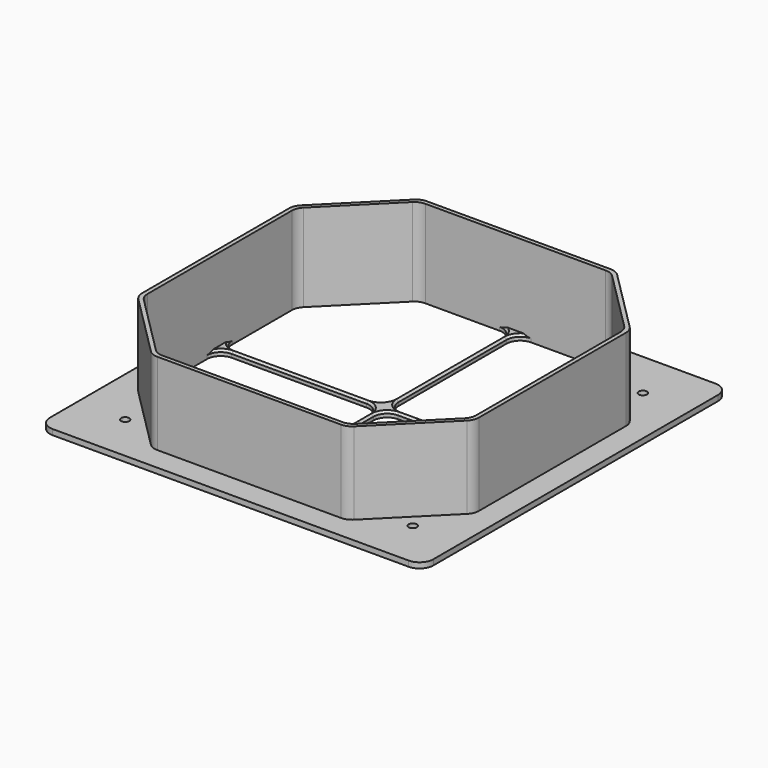
from build123d import *

# Parameters (mm, degrees)
F0_W         = 59.25
F0_H         = 1.5
F0_W_2       = 1.5
F0_H_2       = 59.25
F1_DEPTH     = 2
F0_W_3       = 140
F0_H_3       = 140
F2_DEPTH     = 32
F3_D         = 3
F4_R         = 5
F5_T1_DEPTH  = 49.25
F5_T3_DEPTH  = 49.25
F5_T5_DEPTH  = 49.25
F5_T7_DEPTH  = 49.25
F5_T12_ANGLE = 127.5884718038
F5_T15_ANGLE = 90
F5_T19_ANGLE = 127.5884718038
F5_T24_ANGLE = 127.5884718038
F5_T27_ANGLE = 90
F5_T31_ANGLE = 127.5884718038
F5_T36_ANGLE = 127.5884718038
F5_T39_ANGLE = 90
F5_T43_ANGLE = 127.5884718038
F5_T48_ANGLE = 127.5884718038
F5_T53_ANGLE = 127.5884718038
F5_T56_ANGLE = 90


# Not quite as in the source:
# - a fillet or chamfer that OpenCascade refuses, or shapes differently, is made with other operations: its cross-section is extruded or revolved along the edge and cut away or added


with BuildPart() as f1:
    # F0 (on Top) → F1 (new body)
    with BuildSketch(Plane.XY):
        with Locations((-36.375, 0)):
            Rectangle(F0_W, F0_H)
        with Locations((-6, 30.375)):
            Rectangle(F0_W_2, F0_H_2)
        with Locations((-6, -30.375)):
            Rectangle(F0_W_2, F0_H_2)
        with Locations((24.375, 0)):
            Rectangle(F0_W, F0_H)
        with Locations((-6, 0)):
            Rectangle(F0_W_2, F0_H)
    extrude(amount=F1_DEPTH)



with BuildPart() as f1b:
    # F0 (on Top) → F1, piece 2 (new body)
    with BuildSketch(Plane.XY):
        with Locations((-6, 0)):
            Rectangle(F0_W_3, F0_H_3)
        Polygon((55.5000009226, -35.6213207257), (29.6213207257, -61.5000009226), (-41.6213207257, -61.5000009226), (-67.5000009226, -35.6213207257), (-67.5000009226, 35.6213207257), (-41.6213207257, 61.5000009226), (29.6213207257, 61.5000009226), (55.5000009226, 35.6213207257), align=None, mode=Mode.SUBTRACT)
    extrude(amount=F1_DEPTH)


with BuildPart() as f1_1:
    add(f1.part)

    add(f1b.part)  # F2 merges F1b
    # F0 (on Top) → F2 (join)
    with BuildSketch(Plane.XY):
        Polygon((-41.6213207257, -61.5000009226), (29.6213207257, -61.5000009226), (55.5000009226, -35.6213207257), (55.5000009226, 35.6213207257), (29.6213207257, 61.5000009226), (-41.6213207257, 61.5000009226), (-67.5000009226, 35.6213207257), (-67.5000009226, -35.6213207257), align=None)
        Polygon((29, 60), (54, 35), (54, 0.75), (54, -0.75), (54, -35), (29, -60), (-5.25, -60), (-6.75, -60), (-41, -60), (-66, -35), (-66, -0.75), (-66, 0.75), (-66, 35), (-41, 60), (-6.75, 60), (-5.25, 60), align=None, mode=Mode.SUBTRACT)
    extrude(amount=F2_DEPTH)

    # F3 (through all)
    with Locations(Plane(origin=(0, 0, 0), x_dir=(1, 0, 0), z_dir=(0, 0, -1))):
        with Locations((-58.5, -52.5), (-58.5, 52.5), (46.5, 52.5), (46.5, -52.5)):
            Hole(F3_D / 2)

    # F4
    f4_edges = [f1_1.edges().sort_by_distance(p)[0] for p in [
        (-6.75, 60, 1),
        (-6.75, 0.75, 1),
        (-41, 60, 16),
        (-66, 35, 16),
        (-66, -0.75, 1),
        (-66, 0.75, 1),
        (-66, -35, 16),
        (-6.75, -0.75, 1),
        (-6.75, -60, 1),
        (29, -60, 16),
        (54, -35, 16),
        (54, -0.75, 1),
        (-5.25, -0.75, 1),
        (-5.25, -60, 1),
        (29, 60, 16),
        (54, 35, 16),
        (54, 0.75, 1),
        (-5.25, 0.75, 1),
        (-5.25, 60, 1),
        (-41, -60, 16),
        (-76, -70, 1),
        (64, -70, 1),
        (64, 70, 1),
        (-76, 70, 1),
        (-67.500001, -35.621321, 17),
        (-41.621321, -61.500001, 17),
        (29.621321, -61.500001, 17),
        (55.500001, -35.621321, 17),
        (55.500001, 35.621321, 17),
        (29.621321, 61.500001, 17),
        (-41.621321, 61.500001, 17),
        (-67.500001, 35.621321, 17),
    ]]
    fillet(f4_edges, radius=F4_R)

    # F5: chamfer of 0.75 on 20 edges, made by hand

    # F5_s2 → F5_t1 (cut)
    with BuildSketch(Plane.YZ.offset(-61)):
        Polygon((-0.75, 1.25), (0, 2), (-0.75, 2), align=None)
        Polygon((0.75, 1.25), (0, 2), (0.75, 2), align=None)
    extrude(amount=F5_T1_DEPTH, mode=Mode.SUBTRACT)

    # F5_s4 → F5_t3 (cut)
    with BuildSketch(Plane.YZ.offset(-0.25)):
        Polygon((-0.75, 1.25), (0, 2), (-0.75, 2), align=None)
        Polygon((0.75, 1.25), (0, 2), (0.75, 2), align=None)
    extrude(amount=F5_T3_DEPTH, mode=Mode.SUBTRACT)

    # F5_s6 → F5_t5 (cut)
    with BuildSketch(Plane.XZ.offset(-55)):
        Polygon((-5.25, 1.25), (-6, 2), (-5.25, 2), align=None)
        Polygon((-6.75, 1.25), (-6, 2), (-6.75, 2), align=None)
    extrude(amount=F5_T5_DEPTH, mode=Mode.SUBTRACT)

    # F5_s8 → F5_t7 (cut)
    with BuildSketch(Plane.XZ.offset(5.75)):
        Polygon((-6.75, 1.25), (-6, 2), (-6.75, 2), align=None)
        Polygon((-5.25, 1.25), (-6, 2), (-5.25, 2), align=None)
    extrude(amount=F5_T7_DEPTH, mode=Mode.SUBTRACT)


with BuildPart() as f5_tool10:
    # F5_s11 → F5_t12 (revolve)
    with BuildSketch(Plane(origin=(-19.9177172188, 25.8744507102, 0), x_dir=(0, 0, 1), z_dir=(0.6099857389, -0.7924123916, 0))):
        Polygon((1.25, 56.8445738842), (2, 57.5945738842), (2, 56.8445738842), align=None)
    revolve(axis=Axis((-61, -5.75, 2), (0, 0, -1)), revolution_arc=F5_T12_ANGLE)

    split(bisect_by=Plane.YZ.offset(-66), keep=Keep.TOP)


with BuildPart() as f1_2:
    add(f1_1.part)

    # F5_t9: cut F5_tool10
    add(f5_tool10.part, mode=Mode.SUBTRACT)

    # F5_s14 → F5_t15 (revolve, cut)
    with BuildSketch(Plane.YZ.offset(-11.75)):
        Polygon((-0.75, 1.25), (0, 2), (-0.75, 2), align=None)
    revolve(axis=Axis((-11.75, -5.75, 2), (0, 0, -1)), revolution_arc=F5_T15_ANGLE, mode=Mode.SUBTRACT)


with BuildPart() as f5_tool17:
    # F5_s18 → F5_t19 (revolve)
    with BuildSketch(Plane(origin=(19.2067847712, -14.7850600594, 0), x_dir=(0, 0, 1), z_dir=(-0.7924123916, 0.6099857389, 0))):
        Polygon((1.25, -55.7500139684), (2, -56.5000139684), (2, -55.7500139684), align=None)
    revolve(axis=Axis((-11.75, -55, 2), (0, 0, 1)), revolution_arc=F5_T19_ANGLE)

    split(bisect_by=Plane.XZ.offset(60), keep=Keep.BOTTOM)


with BuildPart() as f1_3:
    add(f1_2.part)

    # F5_t16: cut F5_tool17
    add(f5_tool17.part, mode=Mode.SUBTRACT)


with BuildPart() as f5_tool22:
    # F5_s23 → F5_t24 (revolve)
    with BuildSketch(Plane(origin=(15.4527259985, 20.0741276118, 0), x_dir=(0, 0, 1), z_dir=(-0.6099857389, -0.7924123916, 0))):
        Polygon((1.25, -47.3356251854), (2, -48.0856251854), (2, -47.3356251854), align=None)
    revolve(axis=Axis((49, -5.75, 2), (0, 0, 1)), revolution_arc=F5_T24_ANGLE)

    split(bisect_by=Plane.YZ.offset(54), keep=Keep.BOTTOM)


with BuildPart() as f1_4:
    add(f1_3.part)

    # F5_t21: cut F5_tool22
    add(f5_tool22.part, mode=Mode.SUBTRACT)

    # F5_s26 → F5_t27 (revolve, cut)
    with BuildSketch(Plane.YZ.offset(-0.25)):
        Polygon((-0.75, 1.25), (0, 2), (-0.75, 2), align=None)
    revolve(axis=Axis((-0.25, -5.75, 2), (0, 0, 1)), revolution_arc=F5_T27_ANGLE, mode=Mode.SUBTRACT)


with BuildPart() as f5_tool29:
    # F5_s30 → F5_t31 (revolve)
    with BuildSketch(Plane(origin=(-26.7417935508, -20.5853831579, 0), x_dir=(0, 0, 1), z_dir=(0.7924123916, 0.6099857389, 0))):
        Polygon((1.25, 48.4301851013), (2, 49.1801851013), (2, 48.4301851013), align=None)
    revolve(axis=Axis((-0.25, -55, 2), (0, 0, -1)), revolution_arc=F5_T31_ANGLE)

    split(bisect_by=Plane.XZ.offset(60), keep=Keep.BOTTOM)


with BuildPart() as f1_5:
    add(f1_4.part)

    # F5_t28: cut F5_tool29
    add(f5_tool29.part, mode=Mode.SUBTRACT)


with BuildPart() as f5_tool34:
    # F5_s35 → F5_t36 (revolve)
    with BuildSketch(Plane(origin=(19.2067847712, 14.7850600594, 0), x_dir=(0, 0, 1), z_dir=(-0.7924123916, -0.6099857389, 0))):
        Polygon((1.25, 55.7500139684), (2, 56.5000139684), (2, 55.7500139684), align=None)
    revolve(axis=Axis((-11.75, 55, 2), (0, 0, -1)), revolution_arc=F5_T36_ANGLE)

    split(bisect_by=Plane.XZ.offset(-60), keep=Keep.TOP)


with BuildPart() as f1_6:
    add(f1_5.part)

    # F5_t33: cut F5_tool34
    add(f5_tool34.part, mode=Mode.SUBTRACT)

    # F5_s38 → F5_t39 (revolve, cut)
    with BuildSketch(Plane.XZ.offset(-5.75)):
        Polygon((-6.75, 1.25), (-6, 2), (-6.75, 2), align=None)
    revolve(axis=Axis((-11.75, 5.75, 2), (0, 0, -1)), revolution_arc=F5_T39_ANGLE, mode=Mode.SUBTRACT)


with BuildPart() as f5_tool41:
    # F5_s42 → F5_t43 (revolve)
    with BuildSketch(Plane(origin=(-19.9177172188, -25.8744507102, 0), x_dir=(0, 0, 1), z_dir=(0.6099857389, 0.7924123916, 0))):
        Polygon((1.25, -56.8445738842), (2, -57.5945738842), (2, -56.8445738842), align=None)
    revolve(axis=Axis((-61, 5.75, 2), (0, 0, 1)), revolution_arc=F5_T43_ANGLE)

    split(bisect_by=Plane.YZ.offset(-66), keep=Keep.TOP)


with BuildPart() as f1_7:
    add(f1_6.part)

    # F5_t40: cut F5_tool41
    add(f5_tool41.part, mode=Mode.SUBTRACT)


with BuildPart() as f5_tool46:
    # F5_s47 → F5_t48 (revolve)
    with BuildSketch(Plane(origin=(-26.7417935508, 20.5853831579, 0), x_dir=(0, 0, 1), z_dir=(0.7924123916, -0.6099857389, 0))):
        Polygon((1.25, -48.4301851013), (2, -49.1801851013), (2, -48.4301851013), align=None)
    revolve(axis=Axis((-0.25, 55, 2), (0, 0, 1)), revolution_arc=F5_T48_ANGLE)

    split(bisect_by=Plane.XZ.offset(-60), keep=Keep.TOP)


with BuildPart() as f1_8:
    add(f1_7.part)

    # F5_t45: cut F5_tool46
    add(f5_tool46.part, mode=Mode.SUBTRACT)


with BuildPart() as f5_tool51:
    # F5_s52 → F5_t53 (revolve)
    with BuildSketch(Plane(origin=(15.4527259985, -20.0741276118, 0), x_dir=(0, 0, 1), z_dir=(-0.6099857389, 0.7924123916, 0))):
        Polygon((1.25, 47.3356251854), (2, 48.0856251854), (2, 47.3356251854), align=None)
    revolve(axis=Axis((49, 5.75, 2), (0, 0, -1)), revolution_arc=F5_T53_ANGLE)

    split(bisect_by=Plane.YZ.offset(54), keep=Keep.BOTTOM)


with BuildPart() as f1_9:
    add(f1_8.part)

    # F5_t50: cut F5_tool51
    add(f5_tool51.part, mode=Mode.SUBTRACT)

    # F5_s55 → F5_t56 (revolve, cut)
    with BuildSketch(Plane.XZ.offset(-5.75)):
        Polygon((-5.25, 1.25), (-6, 2), (-5.25, 2), align=None)
    revolve(axis=Axis((-0.25, 5.75, 2), (0, 0, 1)), revolution_arc=F5_T56_ANGLE, mode=Mode.SUBTRACT)


solid = f1_9.part
